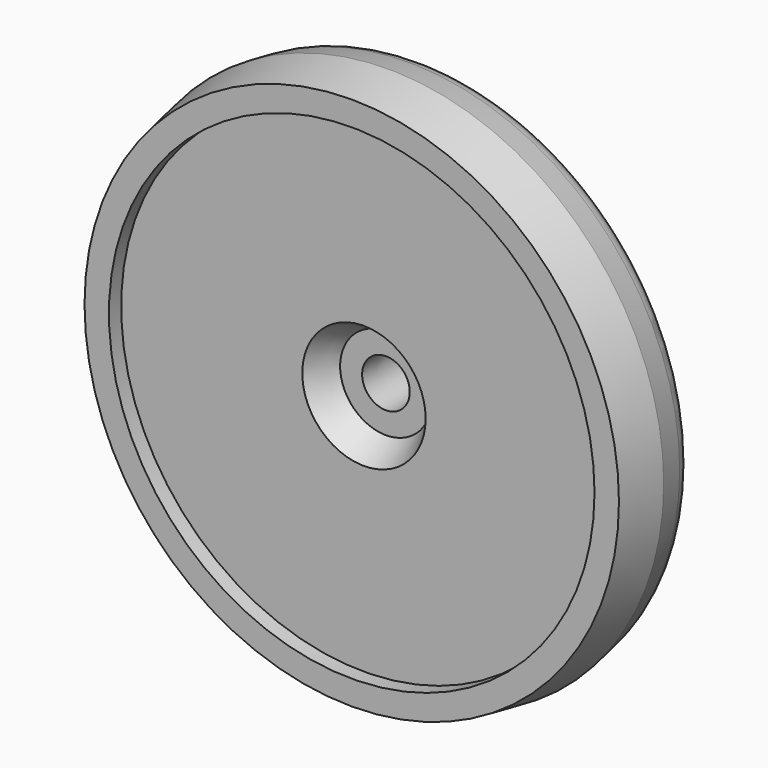
from build123d import *

# Parameters (mm, degrees)
F2_R    = 3.81
F3_R    = 2.032
F4_R    = 0.508
F5_SIZE = 0.508


# Not quite as in the source:
# - two fillets or chamfers of one size are made in one step


with BuildPart() as f1:
    # F0 (on Top) → F1 (revolve)
    with BuildSketch(Plane.XY):
        Polygon((4.064, 11.684), (1.905, 11.684), (1.905, 7.874), (1.9803709704, 3.556), (3.81, 3.556), (5.1298227154, 1.27), (20.193, 1.27), (20.193, 0), (22.225, 0), (22.8968057965, 3.81), (22.225, 7.62), (11.7266037172, 7.62), (11.176, 15.494), (8.44037432, 15.494), (8.44037432, 9.6999123219), (7.17037432, 9.6999123219), (6.985, 20.32), (4.2147419407, 20.32), align=None)
    revolve(axis=Axis((0, 28.982443735, 0), (0, 1, 0)))

    # F2
    f2_edges = [f1.edges().sort_by_distance(p)[0] for p in [
        (-11.726604, 7.62, 0),
    ]]
    fillet(f2_edges, radius=F2_R)

    # F3
    f3_edges = [f1.edges().sort_by_distance(p)[0] for p in [
        (-22.225, 7.62, 0),
    ]]
    fillet(f3_edges, radius=F3_R)

    # F4
    f4_edges = [f1.edges().sort_by_distance(p)[0] for p in [
        (-8.440374, 9.699912, 0),
        (-7.170374, 9.699912, 0),
        (-4.214742, 20.32, 0),
    ]]
    fillet(f4_edges, radius=F4_R)

    # F5
    f5_edges = [f1.edges().sort_by_distance(p)[0] for p in [
        (-11.176, 15.494, 0),
    ]]
    chamfer(f5_edges, length=F5_SIZE)


solid = f1.part
